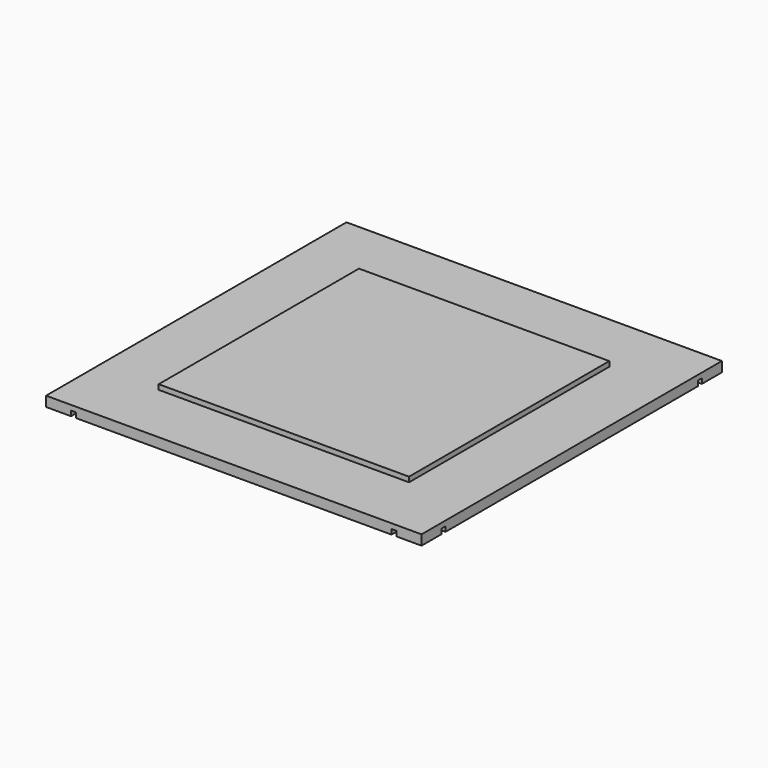
from build123d import *

# Parameters (mm, degrees)
F0_W     = 75
F0_H     = 75
F0_W_2   = 50
F0_H_2   = 50
F1_DEPTH = 2
F2_DEPTH = 3
F3_W     = 1
F3_H     = 5
F3_W_2   = 5
F3_H_2   = 1
F3_W_3   = 63
F3_H_3   = 63
F4_DEPTH = 1


with BuildPart() as f1:
    # F0 (on Top) → F1 (new body)
    with BuildSketch(Plane.XY):
        Rectangle(F0_W, F0_H)
        Rectangle(F0_W_2, F0_H_2, mode=Mode.SUBTRACT)
        Rectangle(F0_W_2, F0_H_2)
    extrude(amount=F1_DEPTH)

    # F0 (on Top) → F2 (join)
    with BuildSketch(Plane.XY):
        Rectangle(F0_W_2, F0_H_2)
    extrude(amount=F2_DEPTH)

    # F3 (on face) → F4 (cut)
    with BuildSketch(Plane.XY):
        with Locations((-32, -35)):
            Rectangle(F3_W, F3_H)
        with Locations((-35, -32)):
            Rectangle(F3_W_2, F3_H_2)
        with Locations((-32, -32)):
            Rectangle(F3_W, F3_H_2)
        with Locations((0, -32)):
            Rectangle(F3_W_3, F3_H_2)
        with Locations((-32, 0)):
            Rectangle(F3_W, F3_H_3)
        with Locations((32, -32)):
            Rectangle(F3_W, F3_H_2)
        with Locations((32, -35)):
            Rectangle(F3_W, F3_H)
        with Locations((-35, 32)):
            Rectangle(F3_W_2, F3_H_2)
        with Locations((-32, 32)):
            Rectangle(F3_W, F3_H_2)
        with Locations((0, 32)):
            Rectangle(F3_W_3, F3_H_2)
        with Locations((32, 0)):
            Rectangle(F3_W, F3_H_3)
        with Locations((35, -32)):
            Rectangle(F3_W_2, F3_H_2)
        with Locations((-32, 35)):
            Rectangle(F3_W, F3_H)
        with Locations((32, 32)):
            Rectangle(F3_W, F3_H_2)
        with Locations((32, 35)):
            Rectangle(F3_W, F3_H)
        with Locations((35, 32)):
            Rectangle(F3_W_2, F3_H_2)
    extrude(amount=F4_DEPTH, mode=Mode.SUBTRACT)


solid = f1.part
